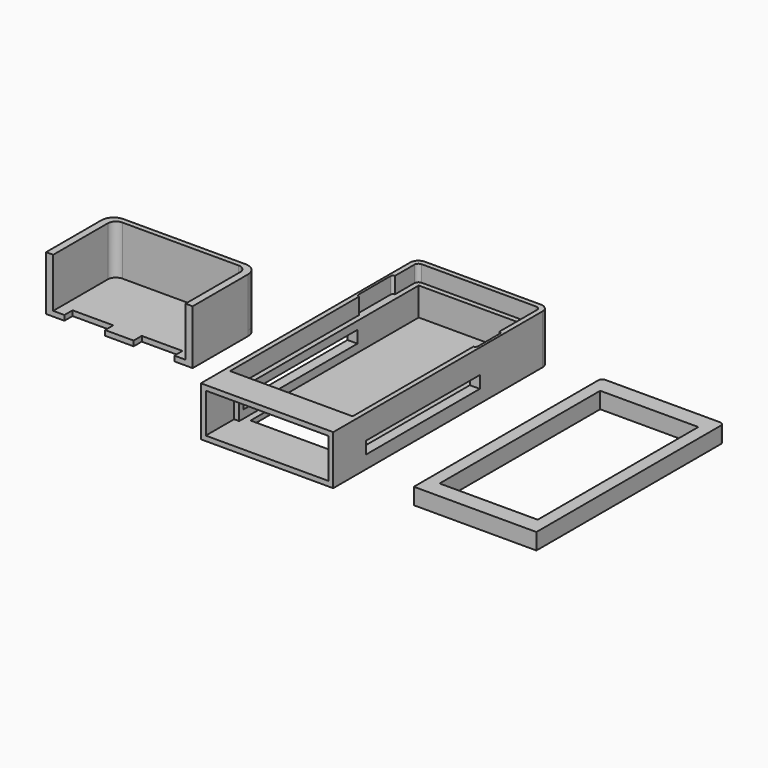
from build123d import *

# Parameters (mm, degrees)
F0_W      = 82.55
F0_H      = 152.4
F0_W_2    = 62.23
F0_H_2    = 16.1877755683
F1_DEPTH  = 30.7975
F2_W      = 76.454
F2_H      = 146.304
F2_W_2    = 62.23
F2_H_2    = 16.1877755683
F3_DEPTH  = 10.16
F4_W      = 70.104
F4_H      = 139.954
F4_W_2    = 62.23
F4_H_2    = 16.1877755683
F5_DEPTH  = 17.5895
F0_H_3    = 15.875
F6_DEPTH  = 30.7975
F7_W      = 76.454
F7_H      = 24.7015
F8_DEPTH  = 22.098
F9_W      = 88.9
F9_H      = 7.62
F10_DEPTH = 82.55
F11_R     = 5.08
F12_W     = 27.94
F12_H     = 10.16
F13_DEPTH = 1.524
F14_R     = 1.52399
F15_W     = 20.32
F15_H     = 10.16
F16_DEPTH = 1.524
F17_R     = 1.52399
F18_R     = 2.54
F20_DEPTH = 3.175
F21_R     = 7.62
F23_DEPTH = 30.7975
F24_R     = 5.08
F25_W     = 76.454
F25_H     = 146.304
F25_W_2   = 61.214
F25_H_2   = 125.222
F26_DEPTH = 10.16
F27_R     = 2.54


# Not quite as in the source:
# - a fillet or chamfer is up to 0.001 mm smaller than in the source, because OpenCascade refuses the exact size


with BuildPart() as f1:
    # F0 (on Top) → F1 (new body)
    with BuildSketch(Plane.XY):
        with Locations((-4.5213731422, -3.2830588596)):
            Rectangle(F0_W, F0_H)
        with Locations((-4.5213731422, -61.2291710755)):
            Rectangle(F0_W_2, F0_H_2, mode=Mode.SUBTRACT)
    extrude(amount=F1_DEPTH)

    # F2 (on face) → F3 (cut)
    with BuildSketch(Plane.XY.offset(30.7975)):
        with Locations((-4.5213731422, -3.2830588596)):
            Rectangle(F2_W, F2_H)
        with Locations((-4.5213731422, -61.2291710755)):
            Rectangle(F2_W_2, F2_H_2, mode=Mode.SUBTRACT)
    extrude(amount=-F3_DEPTH, mode=Mode.SUBTRACT)

    # F4 (on face) → F5 (cut)
    with BuildSketch(Plane.XY.offset(20.6375)):
        with Locations((-4.5213731422, -3.2830588596)):
            Rectangle(F4_W, F4_H)
        with Locations((-4.5213731422, -61.2291710755)):
            Rectangle(F4_W_2, F4_H_2, mode=Mode.SUBTRACT)
    extrude(amount=-F5_DEPTH, mode=Mode.SUBTRACT)

    # F0 (on Top) → F6 (join)
    with BuildSketch(Plane.XY):
        with Locations((-4.5213731422, -87.4205588596)):
            Rectangle(F0_W, F0_H_3)
    extrude(amount=F6_DEPTH)

    # F7 (on face) → F8 (cut, through all)
    with BuildSketch(Plane.XZ.offset(95.3580588596)):
        with Locations((-4.5213731422, 15.39875)):
            Rectangle(F7_W, F7_H)
    extrude(amount=-F8_DEPTH, mode=Mode.SUBTRACT)

    # F9 (on face) → F10 (cut, through all)
    with BuildSketch(Plane(origin=(-45.7963731422, 0, 0), x_dir=(0, -1, 0), z_dir=(-1, 0, 0))):
        with Locations((25.5080588596, 11.90625)):
            Rectangle(F9_W, F9_H)
    extrude(amount=-F10_DEPTH, mode=Mode.SUBTRACT)

    # F11
    f11_edges = [f1.edges().sort_by_distance(p)[0] for p in [
        (-45.796373, 72.916941, 15.39875),
        (36.753627, 72.916941, 15.39875),
    ]]
    fillet(f11_edges, radius=F11_R)

    # F12 (on face) → F13 (cut)
    with BuildSketch(Plane.YZ.offset(-42.7483731422)):
        with Locations((38.1189411404, 25.7175)):
            Rectangle(F12_W, F12_H)
    extrude(amount=-F13_DEPTH, mode=Mode.SUBTRACT)

    # F14 (radius 1.524 in the source; OpenCascade refuses exactly that, so slightly less here)
    f14_edges = [f1.edges().sort_by_distance(p)[0] for p in [
        (-44.272373, 52.088941, 25.7175),
        (-44.272373, 24.148941, 25.7175),
    ]]
    fillet(f14_edges, radius=F14_R)

    # F15 (on face) → F16 (cut)
    with BuildSketch(Plane(origin=(33.7056268578, 0, 0), x_dir=(0, -1, 0), z_dir=(-1, 0, 0))):
        with Locations((-27.9589411404, 25.7175)):
            Rectangle(F15_W, F15_H)
    extrude(amount=-F16_DEPTH, mode=Mode.SUBTRACT)

    # F17 (radius 1.524 in the source; OpenCascade refuses exactly that, so slightly less here)
    f17_edges = [f1.edges().sort_by_distance(p)[0] for p in [
        (35.229627, 38.118941, 25.7175),
        (35.229627, 17.798941, 25.7175),
    ]]
    fillet(f17_edges, radius=F17_R)

    # F18
    f18_edges = [f1.edges().sort_by_distance(p)[0] for p in [
        (-42.748373, 69.868941, 25.7175),
        (33.705627, 69.868941, 25.7175),
    ]]
    fillet(f18_edges, radius=F18_R)


with BuildPart() as f20:
    # F19 (on Top) → F20 (new body)
    with BuildSketch(Plane.XY):
        Polygon((-95.8238354015, 11.5645605006), (-187.2638354015, 11.5645605006), (-187.2638354015, -39.2354394994), (-175.8338354015, -39.2354394994), (-175.8338354015, -32.8854394994), (-150.4338354015, -32.8854394994), (-150.4338354015, -39.2354394994), (-132.6538354015, -39.2354394994), (-132.6538354015, -32.8854394994), (-107.2538354015, -32.8854394994), (-107.2538354015, -39.2354394994), (-95.8238354015, -39.2354394994), align=None)
    extrude(amount=F20_DEPTH)

    # F21
    f21_edges = [f20.edges().sort_by_distance(p)[0] for p in [
        (-187.263835, 11.564561, 1.5875),
        (-95.823835, 11.564561, 1.5875),
    ]]
    fillet(f21_edges, radius=F21_R)

    # F22 (on face) → F23 (join)
    with BuildSketch(Plane.XY.offset(3.175)):
        with BuildLine():
            Line((-182.8188354015, -39.2354394994), (-182.8188354015, 8.3895605006))
            Line((-182.8188354015, 8.3895605006), (-100.2688354015, 8.3895605006))
            Line((-100.2688354015, 8.3895605006), (-100.2688354015, -39.2354394994))
            Line((-100.2688354015, -39.2354394994), (-95.8238354015, -39.2354394994))
            Line((-95.8238354015, -39.2354394994), (-95.8238354015, 3.9445605006))
            ThreePointArc((-95.8238354015, 3.9445605006), (-98.0556817289, 9.3327141732), (-103.4438354015, 11.5645605006))
            Line((-103.4438354015, 11.5645605006), (-179.6438354015, 11.5645605006))
            ThreePointArc((-179.6438354015, 11.5645605006), (-185.0319890742, 9.3327141732), (-187.2638354015, 3.9445605006))
            Line((-187.2638354015, 3.9445605006), (-187.2638354015, -39.2354394994))
            Line((-187.2638354015, -39.2354394994), (-182.8188354015, -39.2354394994))
        make_face()
    extrude(amount=F23_DEPTH)

    # F24
    f24_edges = [f20.edges().sort_by_distance(p)[0] for p in [
        (-182.818835, 8.389561, 18.57375),
        (-100.268835, 8.389561, 18.57375),
    ]]
    fillet(f24_edges, radius=F24_R)


with BuildPart() as f26:
    # F25 (on Top) → F26 (new body)
    with BuildSketch(Plane.XY):
        with Locations((116.8624450643, -11.695331095)):
            Rectangle(F25_W, F25_H)
        with Locations((116.8624450643, -11.695331095)):
            Rectangle(F25_W_2, F25_H_2, mode=Mode.SUBTRACT)
    extrude(amount=F26_DEPTH)

    # F27
    f27_edges = [f26.edges().sort_by_distance(p)[0] for p in [
        (78.635445, 61.456669, 5.08),
        (155.089445, 61.456669, 5.08),
    ]]
    fillet(f27_edges, radius=F27_R)


solid = Compound([f1.part, f20.part, f26.part])
